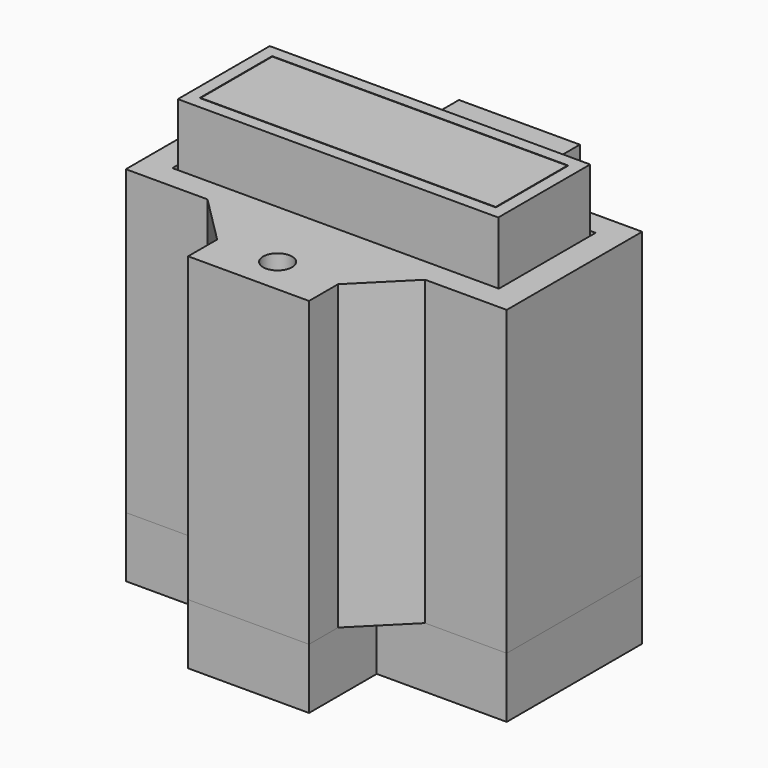
from build123d import *

# Parameters (mm, degrees)
F0_W      = 26.5
F0_H      = 9.5
F1_DEPTH  = 13
F2_W      = 26.5
F2_H      = 9.5
F2_W_2    = 24.5
F2_H_2    = 7.5
F3_DEPTH  = 6
F4_W      = 1
F4_H      = 7.5
F5_DEPTH  = 4
F6_R      = 3.1
F7_DEPTH  = 19
F8_W      = 1.5
F8_H      = 9.5
F9_DEPTH  = 9
F10_R     = 2.55
F11_DEPTH = 3
F13_W     = 27
F13_H     = 10
F13_W_2   = 10
F13_H_2   = 7
F14_DEPTH = 25
F15_W     = 30
F15_H     = 10
F16_DEPTH = 20
F17_R     = 1.2
F18_DEPTH = 25
F19_W     = 5
F19_H     = 5
F19_R     = 4
F19_W_2   = 10
F19_H_2   = 7
F19_R_2   = 1.5
F20_DEPTH = 5
F21_SIZE  = 4
F23_W     = 5
F23_H     = 9
F24_DEPTH = 11.5
F25_W     = 24.4
F25_H     = 7.4
F26_DEPTH = 2


with BuildPart() as f1:
    # F0 (on Top) → F1 (new body)
    with BuildSketch(Plane.XY):
        Rectangle(F0_W, F0_H)
    extrude(amount=F1_DEPTH)

    # F2 (on face) → F3 (join)
    with BuildSketch(Plane.XY.offset(13)):
        Rectangle(F2_W, F2_H)
        Rectangle(F2_W_2, F2_H_2, mode=Mode.SUBTRACT)
    extrude(amount=F3_DEPTH)

    # F4 (on face) → F5 (join)
    with BuildSketch(Plane.XY.offset(13)):
        with Locations((-11.75, 0)):
            Rectangle(F4_W, F4_H)
        with Locations((11.75, 0)):
            Rectangle(F4_W, F4_H)
    extrude(amount=F5_DEPTH)

    # F6 (on face) → F7 (cut)
    with BuildSketch(Plane.XY.offset(13)):
        with Locations((-6.5, 0)):
            Circle(F6_R)
        with Locations((6.5, 0)):
            Circle(F6_R)
    extrude(amount=-F7_DEPTH, mode=Mode.SUBTRACT)

    # F8 (on face) → F9 (join)
    with BuildSketch(Plane(origin=(0, 0, 0), x_dir=(1, 0, 0), z_dir=(0, 0, -1))):
        with Locations((-14, 0)):
            Rectangle(F8_W, F8_H)
        with Locations((14, 0)):
            Rectangle(F8_W, F8_H)
    extrude(amount=-F9_DEPTH)

    # F10 (on face) → F11 (cut)
    with BuildSketch(Plane(origin=(0, 0, 0), x_dir=(1, 0, 0), z_dir=(0, 0, -1))):
        Circle(F10_R)
    extrude(amount=-F11_DEPTH, mode=Mode.SUBTRACT)


with BuildPart() as f14:
    # F13 (on offset) → F14 (new body)
    with BuildSketch(Plane.XY.offset(14)):
        Polygon((5, -7), (15.75, -7), (15.75, 7), (5, 7), (-5, 7), (-15.75, 7), (-15.75, -7), (-5, -7), align=None)
        Rectangle(F13_W, F13_H, mode=Mode.SUBTRACT)
        with Locations((0, -10.5)):
            Rectangle(F13_W_2, F13_H_2)
        with Locations((0, 10.5)):
            Rectangle(F13_W_2, F13_H_2)
    extrude(amount=-F14_DEPTH)

    # F15 (on face) → F16 (cut)
    with BuildSketch(Plane(origin=(0, 0, -11), x_dir=(1, 0, 0), z_dir=(0, 0, -1))):
        Rectangle(F15_W, F15_H)
    extrude(amount=-F16_DEPTH, mode=Mode.SUBTRACT)

    # F17 (on face) → F18 (cut)
    with BuildSketch(Plane.XY.offset(14)):
        with Locations((0, 11)):
            Circle(F17_R)
        with Locations((0, -11)):
            Circle(F17_R)
    extrude(amount=-F18_DEPTH, mode=Mode.SUBTRACT)

    # F21
    f21_edges = [f14.edges().sort_by_distance(p)[0] for p in [
        (-5, 7, 1.5),
        (5, 7, 1.5),
        (5, -7, 1.5),
        (-5, -7, 1.5),
    ]]
    chamfer(f21_edges, length=F21_SIZE)


with BuildPart() as f20:
    # F19 (on face) → F20 (new body)
    with BuildSketch(Plane(origin=(0, 0, -11), x_dir=(1, 0, 0), z_dir=(0, 0, -1))):
        Polygon((5, -7), (15.75, -7), (15.75, 7), (5, 7), (-5, 7), (-15.75, 7), (-15.75, -7), (-5, -7), align=None)
        with Locations((-7.5, 0)):
            Rectangle(F19_W, F19_H, mode=Mode.SUBTRACT)
        Circle(F19_R, mode=Mode.SUBTRACT)
        with Locations((7.5, 0)):
            Rectangle(F19_W, F19_H, mode=Mode.SUBTRACT)
        with Locations((0, -10.5)):
            Rectangle(F19_W_2, F19_H_2)
        with Locations((0, -11)):
            Circle(F19_R_2, mode=Mode.SUBTRACT)
        with Locations((0, 10.5)):
            Rectangle(F19_W_2, F19_H_2)
        with Locations((0, 11)):
            Circle(F19_R_2, mode=Mode.SUBTRACT)
    extrude(amount=F20_DEPTH)


with BuildPart() as f24:
    # F23 (on offset) → F24 (new body)
    with BuildSketch(Plane(origin=(0, 0, -11), x_dir=(1, 0, 0), z_dir=(0, 0, -1))):
        Rectangle(F23_W, F23_H)
    extrude(amount=-F24_DEPTH)


with BuildPart() as f26:
    # F25 (on face) → F26 (new body)
    with BuildSketch(Plane.XY.offset(19)):
        Rectangle(F25_W, F25_H)
    extrude(amount=-F26_DEPTH)


solid = Compound([f1.part, f14.part, f20.part, f24.part, f26.part])
